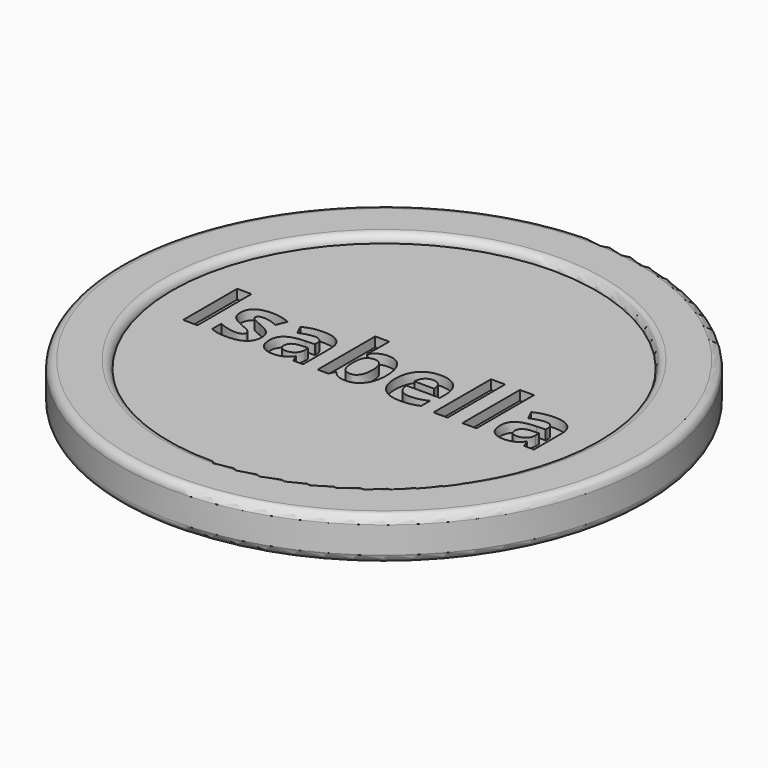
from build123d import *

# Parameters (mm, degrees)
F0_R         = 41.275
F1_DEPTH     = 6.7056
F2_R         = 33.1724
F3_DEPTH     = 1.27
F4_R         = 1.26999
F5_TEXT_SIZE = 14.8068982269
F6_DEPTH     = 1.5
F7_R         = 33.1724
F8_DEPTH     = 1.27


# Not quite as in the source:
# - a fillet or chamfer is up to 0.001 mm smaller than in the source, because OpenCascade refuses the exact size
# - Text() gives the source's letters only with a copy of the font that has no kerning and outlines rounded to 1/6400 em; it was checked with that copy


with BuildPart() as f1:
    # F0 (on Top) → F1 (new body)
    with BuildSketch(Plane.XY):
        Circle(F0_R)
    extrude(amount=F1_DEPTH)

    # F2 (on face) → F3 (cut)
    with BuildSketch(Plane.XY.offset(6.7056)):
        Circle(F2_R)
    extrude(amount=-F3_DEPTH, mode=Mode.SUBTRACT)

    # F4 (radius 1.27 in the source; OpenCascade refuses exactly that, so slightly less here)
    f4_edges = [f1.edges().sort_by_distance(p)[0] for p in [
        (-41.275, 0, 6.7056),
        (-41.275, 0, 0),
        (-33.1724, 0, 6.7056),
    ]]
    fillet(f4_edges, radius=F4_R)

    # F5 (on face) → F6 (cut)
    with BuildSketch(Plane.XY.offset(5.4356)):
        with Locations((-28.575, -5.229807857)):
            Text('Isabella', F5_TEXT_SIZE, font='Open Sans', font_style=FontStyle.BOLD, text_align=(TextAlign.LEFT, TextAlign.BOTTOM))
    extrude(amount=-F6_DEPTH, mode=Mode.SUBTRACT)

    # F7 (on face) → F8 (cut)
    with BuildSketch(Plane(origin=(0, 0, 0), x_dir=(1, 0, 0), z_dir=(0, 0, -1))):
        Circle(F7_R)
    extrude(amount=-F8_DEPTH, mode=Mode.SUBTRACT)


solid = f1.part
